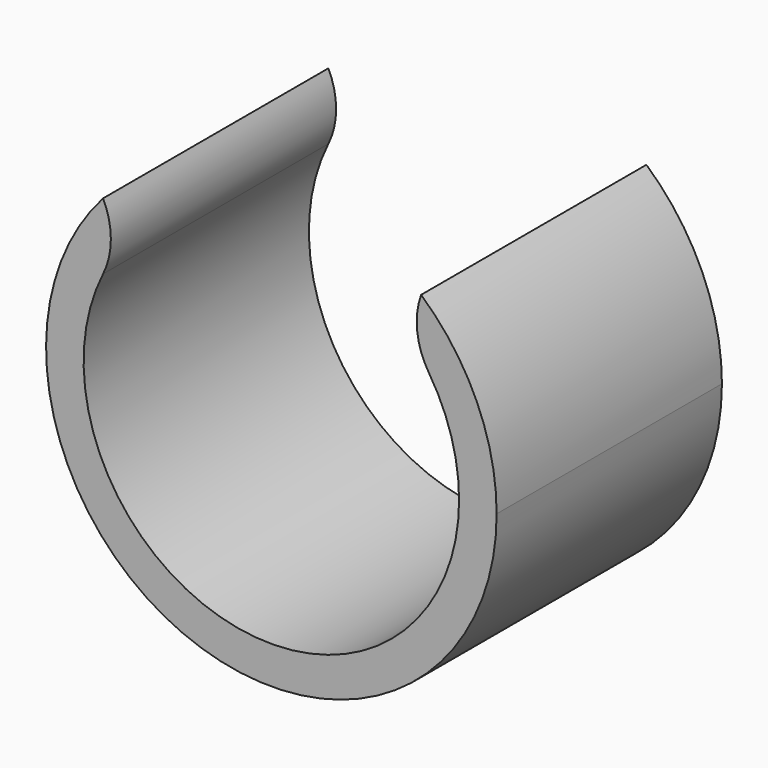
from build123d import *

# Parameters (mm, degrees)
F1_DEPTH    = 19.05
F2_T1_DEPTH = 36.0210888614


# Not quite as in the source:
# - a fillet or chamfer that OpenCascade refuses, or shapes differently, is made with other operations: its cross-section is extruded or revolved along the edge and cut away or added


with BuildPart() as f1:
    # F0 (on Front) → F1 (new body)
    with BuildSketch(Plane.XZ):
        with BuildLine():
            ThreePointArc((8.4433957221, 9.4867838955), (11.5870860373, 5.1989842435), (12.7, 0))
            ThreePointArc((12.7, 0), (-4.5170700973, -11.869544125), (-9.4867838955, 8.4433957221))
            Line((-9.4867838955, 8.4433957221), (-11.3841406746, 10.1320748666))
            ThreePointArc((-11.3841406746, 10.1320748666), (-5.4204841167, -14.24345295), (15.24, 0))
            ThreePointArc((15.24, 0), (13.9045032448, 6.2387810922), (10.1320748666, 11.3841406746))
            Line((10.1320748666, 11.3841406746), (8.4433957221, 9.4867838955))
        make_face()
    extrude(amount=F1_DEPTH)

    # F2: fillet of radius 5.08 on 2 edges, made by hand

    # F2_s2 → F2_t1 (cut)
    with BuildSketch(Plane.XZ.offset(-8.4855444307)):
        with BuildLine():
            ThreePointArc((-11.3843237056, 5.6291361473), (-10.8580531921, 7.8805841193), (-11.3841406746, 10.1320748666))
            Line((-11.3841406746, 10.1320748666), (-9.4867838955, 8.4433957221))
            ThreePointArc((-9.4867838955, 8.4433957221), (-10.5299951264, 7.0999438475), (-11.3843237056, 5.6291361473))
        make_face()
        with BuildLine():
            ThreePointArc((10.6545556025, 6.9116166642), (9.8706902669, 9.0868255644), (10.1320748666, 11.3841406746))
            Line((10.1320748666, 11.3841406746), (8.4433957221, 9.4867838955))
            ThreePointArc((8.4433957221, 9.4867838955), (9.6353934931, 8.2734026998), (10.6545556025, 6.9116166642))
        make_face()
    extrude(amount=F2_T1_DEPTH, mode=Mode.SUBTRACT)


solid = f1.part
